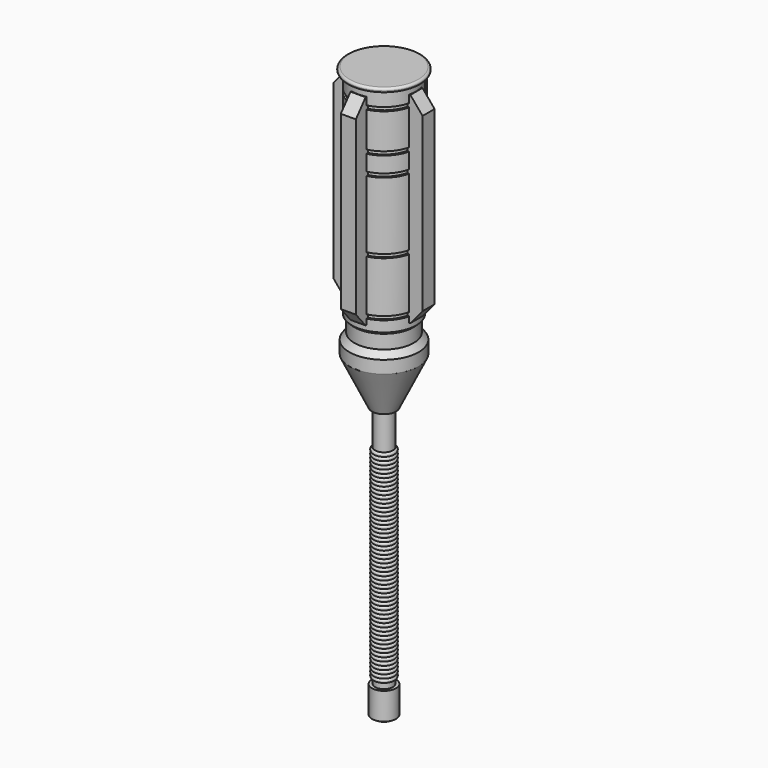
from build123d import *

# Parameters (mm, degrees)
F7_START       = 40
F7_DEPTH       = 31
F10_DEPTH      = 24
F11_COUNT      = 4
F12_R          = 14.2000000015
F13_DEPTH      = 434
F13_DEPTH_BACK = 447.2
F15_START      = -3
F14_R          = 19.2
F14_R_2        = 14.2
F15_DEPTH      = 43
F19_SIZE2      = 4
F19_SIZE       = 4


# Not quite as in the source:
# - ends of sketch curves that miss each other by under 0.0002 mm in the source are joined


with BuildPart() as f2:
    # F0 (on Front) → F2 (revolve)
    with BuildSketch(Plane.XZ):
        Polygon((19.2000000015, -16.7155758262), (55.2000000015, 58.2844241738), (55.2000000015, 78.2844241738), (47.2000000015, 88.5313749398), (47.2000000015, 110.5313749398), (14.2000000015, 110.5313763703), (14.2000000015, -16.7155758262), align=None)
    revolve(axis=Axis((0, 0, 23.2442431152), (0, 0, 1)))


with BuildPart() as f5:
    # F3 (on Front) → F5 (revolve)
    with BuildSketch(Plane.XZ):
        with BuildLine():
            Line((51.2, 112.0996549726), (51.2, 113.5313748121))
            Line((51.2, 113.5313748121), (51.2, 131.5313748121))
            Line((51.2, 131.5313748121), (48.2, 131.5313748121))
            Line((48.2, 131.5313748121), (48.2, 137.5313748121))
            Line((48.2, 137.5313748121), (51.2, 137.5313748121))
            Line((51.2, 137.5313748121), (51.2, 218.5313748121))
            Line((51.2, 218.5313748121), (48.2, 218.5313748121))
            Line((48.2, 218.5313748121), (48.2, 224.5313748121))
            Line((48.2, 224.5313748121), (51.2, 224.5313748121))
            Line((51.2, 224.5313748121), (51.2, 331.5313748121))
            Line((51.2, 331.5313748121), (48.2, 331.5313748121))
            Line((48.2, 331.5313748121), (48.2, 337.5313748121))
            Line((48.2, 337.5313748121), (51.2, 337.5313748121))
            Line((51.2, 337.5313748121), (51.2, 362.5313748121))
            Line((51.2, 362.5313748121), (48.2, 362.5313748121))
            Line((48.2, 362.5313748121), (48.2, 368.5313748121))
            Line((48.2, 368.5313748121), (51.2, 368.5313748121))
            Line((51.2, 368.5313748121), (51.2, 424.5313748121))
            Line((51.2, 424.5313748121), (48.2, 424.5313748121))
            Line((48.2, 424.5313748121), (48.2, 430.5313748121))
            Line((48.2, 430.5313748121), (51.2, 430.5313748121))
            Line((51.2, 430.5313748121), (51.2, 453.5313748121))
            Line((51.2, 453.5313748121), (54.7, 453.5313748121))
            ThreePointArc((54.7, 453.5313748121), (57.1748737342, 454.556501078), (58.2, 457.0313748121))
            ThreePointArc((58.2, 457.0313748121), (57.1748737342, 459.5062485463), (54.7, 460.5313748121))
            Line((54.7, 460.5313748121), (14.2, 460.5313748121))
            Line((14.2, 460.5313748121), (0, 460.5313748121))
            Line((0, 460.5313748121), (0, 430.5313748121))
            Line((0, 430.5313748121), (14.2, 430.5313748121))
            Line((14.2, 430.5313748121), (14.2, 110.5313748121))
            Line((14.2, 110.5313748121), (15.9806390532, 110.5313748121))
            Line((15.9806390532, 110.5313748121), (40.9627765536, 110.5313748121))
            Line((40.9627765536, 110.5313748121), (51.2, 110.5313748121))
            Line((51.2, 110.5313748121), (51.2, 112.0996549726))
        make_face()
    revolve(axis=Axis((0, 0, 255.8234632015), (0, 0, 1)))

    # F19
    f19_edges = [f5.edges().sort_by_distance(p)[0] for p in [
        (-51.2, 0, 110.531375),
    ]]
    chamfer(f19_edges, length=F19_SIZE, length2=F19_SIZE2)


with BuildPart() as f7:
    # F6 (on Front) → F7 (new body)
    with BuildSketch(Plane.XZ.offset(F7_START)):
        Polygon((-12, 122.600607574), (0, 122.600607574), (12, 122.600607574), (12, 442.600607574), (-12, 442.600607574), align=None)
    extrude(amount=F7_DEPTH)

    # F9 (on face) → F10 (cut, through all)
    with BuildSketch(Plane.YZ.offset(12)):
        Polygon((-71, 419.500607574), (-51.6167985198, 442.600607574), (-71, 442.600607574), align=None)
        Polygon((-51.6167985198, 122.600607574), (-71, 145.700607574), (-71, 122.600607574), align=None)
    extrude(amount=-F10_DEPTH, mode=Mode.SUBTRACT)


with BuildPart() as f11_1:
    # F11: instance of F7
    add(f7.part.rotate(Axis((0, 0, 22.6825606078), (0, 0, 1)), 1 * 360 / F11_COUNT))


with BuildPart() as f11_2:
    # F11: instance of F7
    add(f7.part.rotate(Axis((0, 0, 22.6825606078), (0, 0, 1)), 2 * 360 / F11_COUNT))


with BuildPart() as f11_3:
    # F11: instance of F7
    add(f7.part.rotate(Axis((0, 0, 22.6825606078), (0, 0, 1)), 3 * 360 / F11_COUNT))


with BuildPart() as f13:
    # F12 (on face) → F13 (new body, two sides)
    with BuildSketch(Plane(origin=(0, 0, -16.7155758262), x_dir=(1, 0, 0), z_dir=(0, 0, -1))) as f13_sk:
        Circle(F12_R)
    extrude(amount=F13_DEPTH)
    extrude(f13_sk.sketch, amount=-F13_DEPTH_BACK)


with BuildPart() as f15:
    # F14 (on face) → F15 (new body)
    with BuildSketch(Plane(origin=(0, 0, -450.7155758262), x_dir=(1, 0, 0), z_dir=(0, 0, -1)).offset(F15_START)):
        Circle(F14_R)
        Circle(F14_R_2, mode=Mode.SUBTRACT)
    extrude(amount=-F15_DEPTH)


with BuildPart() as f18:
    # F16 (on Right) → F18 (revolve)
    with BuildSketch(Plane.YZ):
        with BuildLine():
            Line((14.2000000924, -78.7955758262), (14.2000000924, -78.8155758262))
            ThreePointArc((14.2000000924, -78.8155758262), (14.3224745795, -78.8130747836), (14.4447448574, -78.8055758262))
            ThreePointArc((14.4447448574, -78.8055758262), (14.3224745795, -78.7980768687), (14.2000000924, -78.7955758262))
        make_face()
        with BuildLine():
            ThreePointArc((14.4447448574, -78.8055758262), (14.3224745795, -78.8130747836), (14.2000000924, -78.8155758262))
            Line((14.2000000924, -78.8155758262), (14.2000000924, -84.7755758262))
            ThreePointArc((14.2000000924, -84.7755758262), (14.3224745795, -84.7780768687), (14.4447448574, -84.7855758262))
            ThreePointArc((14.4447448574, -84.7855758262), (17.2000000924, -81.7955758262), (14.4447448574, -78.8055758262))
        make_face()
        with BuildLine():
            ThreePointArc((14.2000000924, -78.7955758262), (14.3224745795, -78.7980768687), (14.4447448574, -78.8055758262))
            ThreePointArc((14.4447448574, -78.8055758262), (17.1974990499, -75.693101339), (14.2000000924, -72.8155758262))
            Line((14.2000000924, -72.8155758262), (14.2000000924, -78.7955758262))
        make_face()
        with BuildLine():
            ThreePointArc((14.4447448574, -84.7855758262), (14.3224745795, -84.7780768687), (14.2000000924, -84.7755758262))
            Line((14.2000000924, -84.7755758262), (14.2000000924, -84.7955758262))
            ThreePointArc((14.2000000924, -84.7955758262), (14.3224745795, -84.7930747836), (14.4447448574, -84.7855758262))
        make_face()
        with BuildLine():
            ThreePointArc((14.4447448574, -90.7655758262), (17.2000000924, -87.7755758262), (14.4447448574, -84.7855758262))
            ThreePointArc((14.4447448574, -84.7855758262), (14.3224745795, -84.7930747836), (14.2000000924, -84.7955758262))
            Line((14.2000000924, -84.7955758262), (14.2000000924, -90.7555758262))
            ThreePointArc((14.2000000924, -90.7555758262), (14.3224745795, -90.7580768687), (14.4447448574, -90.7655758262))
        make_face()
        with BuildLine():
            ThreePointArc((14.4447448574, -96.7455758262), (17.2000000924, -93.7555758262), (14.4447448574, -90.7655758262))
            ThreePointArc((14.4447448574, -90.7655758262), (14.3224745795, -90.7730747836), (14.2000000924, -90.7755758262))
            Line((14.2000000924, -90.7755758262), (14.2000000924, -96.7355758262))
            ThreePointArc((14.2000000924, -96.7355758262), (14.3224745795, -96.7380768687), (14.4447448574, -96.7455758262))
        make_face()
        with BuildLine():
            ThreePointArc((14.2000000924, -90.7755758262), (14.3224745795, -90.7730747836), (14.4447448574, -90.7655758262))
            ThreePointArc((14.4447448574, -90.7655758262), (14.3224745795, -90.7580768687), (14.2000000924, -90.7555758262))
            Line((14.2000000924, -90.7555758262), (14.2000000924, -90.7755758262))
        make_face()
        with BuildLine():
            ThreePointArc((14.4447448574, -102.7255758262), (17.2000000924, -99.7355758262), (14.4447448574, -96.7455758262))
            ThreePointArc((14.4447448574, -96.7455758262), (14.3224745795, -96.7530747836), (14.2000000924, -96.7555758262))
            Line((14.2000000924, -96.7555758262), (14.2000000924, -102.7155758262))
            ThreePointArc((14.2000000924, -102.7155758262), (14.3224745795, -102.7180768687), (14.4447448574, -102.7255758262))
        make_face()
        with BuildLine():
            ThreePointArc((14.2000000924, -96.7555758262), (14.3224745795, -96.7530747836), (14.4447448574, -96.7455758262))
            ThreePointArc((14.4447448574, -96.7455758262), (14.3224745795, -96.7380768687), (14.2000000924, -96.7355758262))
            Line((14.2000000924, -96.7355758262), (14.2000000924, -96.7555758262))
        make_face()
        with BuildLine():
            ThreePointArc((14.4447448574, -108.7055758262), (17.2000000924, -105.7155758262), (14.4447448574, -102.7255758262))
            ThreePointArc((14.4447448574, -102.7255758262), (14.3224745795, -102.7330747836), (14.2000000924, -102.7355758262))
            Line((14.2000000924, -102.7355758262), (14.2000000924, -108.6955758262))
            ThreePointArc((14.2000000924, -108.6955758262), (14.3224745795, -108.6980768687), (14.4447448574, -108.7055758262))
        make_face()
        with BuildLine():
            ThreePointArc((14.2000000924, -102.7355758262), (14.3224745795, -102.7330747836), (14.4447448574, -102.7255758262))
            ThreePointArc((14.4447448574, -102.7255758262), (14.3224745795, -102.7180768687), (14.2000000924, -102.7155758262))
            Line((14.2000000924, -102.7155758262), (14.2000000924, -102.7355758262))
        make_face()
        with BuildLine():
            ThreePointArc((14.4447448574, -114.6855758262), (17.2000000924, -111.6955758262), (14.4447448574, -108.7055758262))
            ThreePointArc((14.4447448574, -108.7055758262), (14.3224745795, -108.7130747836), (14.2000000924, -108.7155758262))
            Line((14.2000000924, -108.7155758262), (14.2000000924, -114.6755758262))
            ThreePointArc((14.2000000924, -114.6755758262), (14.3224745795, -114.6780768687), (14.4447448574, -114.6855758262))
        make_face()
        with BuildLine():
            ThreePointArc((14.2000000924, -108.7155758262), (14.3224745795, -108.7130747836), (14.4447448574, -108.7055758262))
            ThreePointArc((14.4447448574, -108.7055758262), (14.3224745795, -108.6980768687), (14.2000000924, -108.6955758262))
            Line((14.2000000924, -108.6955758262), (14.2000000924, -108.7155758262))
        make_face()
        with BuildLine():
            ThreePointArc((14.4447448574, -120.6655758262), (17.2000000924, -117.6755758262), (14.4447448574, -114.6855758262))
            ThreePointArc((14.4447448574, -114.6855758262), (14.3224745795, -114.6930747836), (14.2000000924, -114.6955758262))
            Line((14.2000000924, -114.6955758262), (14.2000000924, -120.6555758262))
            ThreePointArc((14.2000000924, -120.6555758262), (14.3224745795, -120.6580768687), (14.4447448574, -120.6655758262))
        make_face()
        with BuildLine():
            ThreePointArc((14.2000000924, -114.6955758262), (14.3224745795, -114.6930747836), (14.4447448574, -114.6855758262))
            ThreePointArc((14.4447448574, -114.6855758262), (14.3224745795, -114.6780768687), (14.2000000924, -114.6755758262))
            Line((14.2000000924, -114.6755758262), (14.2000000924, -114.6955758262))
        make_face()
        with BuildLine():
            ThreePointArc((14.4447448574, -126.6455758262), (17.2000000924, -123.6555758262), (14.4447448574, -120.6655758262))
            ThreePointArc((14.4447448574, -120.6655758262), (14.3224745795, -120.6730747836), (14.2000000924, -120.6755758262))
            Line((14.2000000924, -120.6755758262), (14.2000000924, -126.6355758262))
            ThreePointArc((14.2000000924, -126.6355758262), (14.3224745795, -126.6380768687), (14.4447448574, -126.6455758262))
        make_face()
        with BuildLine():
            ThreePointArc((14.2000000924, -120.6755758262), (14.3224745795, -120.6730747836), (14.4447448574, -120.6655758262))
            ThreePointArc((14.4447448574, -120.6655758262), (14.3224745795, -120.6580768687), (14.2000000924, -120.6555758262))
            Line((14.2000000924, -120.6555758262), (14.2000000924, -120.6755758262))
        make_face()
        with BuildLine():
            ThreePointArc((14.4447448574, -132.6255758262), (17.2000000924, -129.6355758262), (14.4447448574, -126.6455758262))
            ThreePointArc((14.4447448574, -126.6455758262), (14.3224745795, -126.6530747836), (14.2000000924, -126.6555758262))
            Line((14.2000000924, -126.6555758262), (14.2000000924, -132.6155758262))
            ThreePointArc((14.2000000924, -132.6155758262), (14.3224745795, -132.6180768687), (14.4447448574, -132.6255758262))
        make_face()
        with BuildLine():
            ThreePointArc((14.2000000924, -126.6555758262), (14.3224745795, -126.6530747836), (14.4447448574, -126.6455758262))
            ThreePointArc((14.4447448574, -126.6455758262), (14.3224745795, -126.6380768687), (14.2000000924, -126.6355758262))
            Line((14.2000000924, -126.6355758262), (14.2000000924, -126.6555758262))
        make_face()
        with BuildLine():
            ThreePointArc((14.4447448574, -138.6055758262), (17.2000000924, -135.6155758262), (14.4447448574, -132.6255758262))
            ThreePointArc((14.4447448574, -132.6255758262), (14.3224745795, -132.6330747836), (14.2000000924, -132.6355758262))
            Line((14.2000000924, -132.6355758262), (14.2000000924, -138.5955758262))
            ThreePointArc((14.2000000924, -138.5955758262), (14.3224745795, -138.5980768687), (14.4447448574, -138.6055758262))
        make_face()
        with BuildLine():
            ThreePointArc((14.2000000924, -132.6355758262), (14.3224745795, -132.6330747836), (14.4447448574, -132.6255758262))
            ThreePointArc((14.4447448574, -132.6255758262), (14.3224745795, -132.6180768687), (14.2000000924, -132.6155758262))
            Line((14.2000000924, -132.6155758262), (14.2000000924, -132.6355758262))
        make_face()
        with BuildLine():
            ThreePointArc((14.4447448574, -144.5855758262), (17.2000000924, -141.5955758262), (14.4447448574, -138.6055758262))
            ThreePointArc((14.4447448574, -138.6055758262), (14.3224745795, -138.6130747836), (14.2000000924, -138.6155758262))
            Line((14.2000000924, -138.6155758262), (14.2000000924, -144.5755758262))
            ThreePointArc((14.2000000924, -144.5755758262), (14.3224745795, -144.5780768687), (14.4447448574, -144.5855758262))
        make_face()
        with BuildLine():
            ThreePointArc((14.2000000924, -138.6155758262), (14.3224745795, -138.6130747836), (14.4447448574, -138.6055758262))
            ThreePointArc((14.4447448574, -138.6055758262), (14.3224745795, -138.5980768687), (14.2000000924, -138.5955758262))
            Line((14.2000000924, -138.5955758262), (14.2000000924, -138.6155758262))
        make_face()
        with BuildLine():
            ThreePointArc((14.4447448574, -150.5655758262), (17.2000000924, -147.5755758262), (14.4447448574, -144.5855758262))
            ThreePointArc((14.4447448574, -144.5855758262), (14.3224745795, -144.5930747836), (14.2000000924, -144.5955758262))
            Line((14.2000000924, -144.5955758262), (14.2000000924, -150.5555758262))
            ThreePointArc((14.2000000924, -150.5555758262), (14.3224745795, -150.5580768687), (14.4447448574, -150.5655758262))
        make_face()
        with BuildLine():
            ThreePointArc((14.2000000924, -144.5955758262), (14.3224745795, -144.5930747836), (14.4447448574, -144.5855758262))
            ThreePointArc((14.4447448574, -144.5855758262), (14.3224745795, -144.5780768687), (14.2000000924, -144.5755758262))
            Line((14.2000000924, -144.5755758262), (14.2000000924, -144.5955758262))
        make_face()
        with BuildLine():
            ThreePointArc((14.4447448574, -156.5455758262), (17.2000000924, -153.5555758262), (14.4447448574, -150.5655758262))
            ThreePointArc((14.4447448574, -150.5655758262), (14.3224745795, -150.5730747836), (14.2000000924, -150.5755758262))
            Line((14.2000000924, -150.5755758262), (14.2000000924, -156.5355758262))
            ThreePointArc((14.2000000924, -156.5355758262), (14.3224745795, -156.5380768687), (14.4447448574, -156.5455758262))
        make_face()
        with BuildLine():
            ThreePointArc((14.2000000924, -150.5755758262), (14.3224745795, -150.5730747836), (14.4447448574, -150.5655758262))
            ThreePointArc((14.4447448574, -150.5655758262), (14.3224745795, -150.5580768687), (14.2000000924, -150.5555758262))
            Line((14.2000000924, -150.5555758262), (14.2000000924, -150.5755758262))
        make_face()
        with BuildLine():
            ThreePointArc((14.4447448574, -162.5255758262), (17.2000000924, -159.5355758262), (14.4447448574, -156.5455758262))
            ThreePointArc((14.4447448574, -156.5455758262), (14.3224745795, -156.5530747836), (14.2000000924, -156.5555758262))
            Line((14.2000000924, -156.5555758262), (14.2000000924, -162.5155758262))
            ThreePointArc((14.2000000924, -162.5155758262), (14.3224745795, -162.5180768687), (14.4447448574, -162.5255758262))
        make_face()
        with BuildLine():
            ThreePointArc((14.2000000924, -156.5555758262), (14.3224745795, -156.5530747836), (14.4447448574, -156.5455758262))
            ThreePointArc((14.4447448574, -156.5455758262), (14.3224745795, -156.5380768687), (14.2000000924, -156.5355758262))
            Line((14.2000000924, -156.5355758262), (14.2000000924, -156.5555758262))
        make_face()
        with BuildLine():
            ThreePointArc((14.4447448574, -168.5055758262), (17.2000000924, -165.5155758262), (14.4447448574, -162.5255758262))
            ThreePointArc((14.4447448574, -162.5255758262), (14.3224745795, -162.5330747836), (14.2000000924, -162.5355758262))
            Line((14.2000000924, -162.5355758262), (14.2000000924, -168.4955758262))
            ThreePointArc((14.2000000924, -168.4955758262), (14.3224745795, -168.4980768687), (14.4447448574, -168.5055758262))
        make_face()
        with BuildLine():
            ThreePointArc((14.2000000924, -162.5355758262), (14.3224745795, -162.5330747836), (14.4447448574, -162.5255758262))
            ThreePointArc((14.4447448574, -162.5255758262), (14.3224745795, -162.5180768687), (14.2000000924, -162.5155758262))
            Line((14.2000000924, -162.5155758262), (14.2000000924, -162.5355758262))
        make_face()
        with BuildLine():
            ThreePointArc((14.4447448574, -174.4855758262), (17.2000000924, -171.4955758262), (14.4447448574, -168.5055758262))
            ThreePointArc((14.4447448574, -168.5055758262), (14.3224745795, -168.5130747836), (14.2000000924, -168.5155758262))
            Line((14.2000000924, -168.5155758262), (14.2000000924, -174.4755758262))
            ThreePointArc((14.2000000924, -174.4755758262), (14.3224745795, -174.4780768687), (14.4447448574, -174.4855758262))
        make_face()
        with BuildLine():
            ThreePointArc((14.2000000924, -168.5155758262), (14.3224745795, -168.5130747836), (14.4447448574, -168.5055758262))
            ThreePointArc((14.4447448574, -168.5055758262), (14.3224745795, -168.4980768687), (14.2000000924, -168.4955758262))
            Line((14.2000000924, -168.4955758262), (14.2000000924, -168.5155758262))
        make_face()
        with BuildLine():
            ThreePointArc((14.4447448574, -180.4655758262), (17.2000000924, -177.4755758262), (14.4447448574, -174.4855758262))
            ThreePointArc((14.4447448574, -174.4855758262), (14.3224745795, -174.4930747836), (14.2000000924, -174.4955758262))
            Line((14.2000000924, -174.4955758262), (14.2000000924, -180.4555758262))
            ThreePointArc((14.2000000924, -180.4555758262), (14.3224745795, -180.4580768687), (14.4447448574, -180.4655758262))
        make_face()
        with BuildLine():
            ThreePointArc((14.2000000924, -174.4955758262), (14.3224745795, -174.4930747836), (14.4447448574, -174.4855758262))
            ThreePointArc((14.4447448574, -174.4855758262), (14.3224745795, -174.4780768687), (14.2000000924, -174.4755758262))
            Line((14.2000000924, -174.4755758262), (14.2000000924, -174.4955758262))
        make_face()
        with BuildLine():
            ThreePointArc((14.4447448574, -186.4455758262), (17.2000000924, -183.4555758262), (14.4447448574, -180.4655758262))
            ThreePointArc((14.4447448574, -180.4655758262), (14.3224745795, -180.4730747836), (14.2000000924, -180.4755758262))
            Line((14.2000000924, -180.4755758262), (14.2000000924, -186.4355758262))
            ThreePointArc((14.2000000924, -186.4355758262), (14.3224745795, -186.4380768687), (14.4447448574, -186.4455758262))
        make_face()
        with BuildLine():
            ThreePointArc((14.2000000924, -180.4755758262), (14.3224745795, -180.4730747836), (14.4447448574, -180.4655758262))
            ThreePointArc((14.4447448574, -180.4655758262), (14.3224745795, -180.4580768687), (14.2000000924, -180.4555758262))
            Line((14.2000000924, -180.4555758262), (14.2000000924, -180.4755758262))
        make_face()
        with BuildLine():
            ThreePointArc((14.4447448574, -192.4255758262), (17.2000000924, -189.4355758262), (14.4447448574, -186.4455758262))
            ThreePointArc((14.4447448574, -186.4455758262), (14.3224745795, -186.4530747836), (14.2000000924, -186.4555758262))
            Line((14.2000000924, -186.4555758262), (14.2000000924, -192.4155758262))
            ThreePointArc((14.2000000924, -192.4155758262), (14.3224745795, -192.4180768687), (14.4447448574, -192.4255758262))
        make_face()
        with BuildLine():
            ThreePointArc((14.2000000924, -186.4555758262), (14.3224745795, -186.4530747836), (14.4447448574, -186.4455758262))
            ThreePointArc((14.4447448574, -186.4455758262), (14.3224745795, -186.4380768687), (14.2000000924, -186.4355758262))
            Line((14.2000000924, -186.4355758262), (14.2000000924, -186.4555758262))
        make_face()
        with BuildLine():
            ThreePointArc((14.4447448574, -198.4055758262), (17.2000000924, -195.4155758262), (14.4447448574, -192.4255758262))
            ThreePointArc((14.4447448574, -192.4255758262), (14.3224745795, -192.4330747836), (14.2000000924, -192.4355758262))
            Line((14.2000000924, -192.4355758262), (14.2000000924, -198.3955758262))
            ThreePointArc((14.2000000924, -198.3955758262), (14.3224745795, -198.3980768687), (14.4447448574, -198.4055758262))
        make_face()
        with BuildLine():
            ThreePointArc((14.2000000924, -192.4355758262), (14.3224745795, -192.4330747836), (14.4447448574, -192.4255758262))
            ThreePointArc((14.4447448574, -192.4255758262), (14.3224745795, -192.4180768687), (14.2000000924, -192.4155758262))
            Line((14.2000000924, -192.4155758262), (14.2000000924, -192.4355758262))
        make_face()
        with BuildLine():
            ThreePointArc((14.4447448574, -204.3855758262), (17.2000000924, -201.3955758262), (14.4447448574, -198.4055758262))
            ThreePointArc((14.4447448574, -198.4055758262), (14.3224745795, -198.4130747836), (14.2000000924, -198.4155758262))
            Line((14.2000000924, -198.4155758262), (14.2000000924, -204.3755758262))
            ThreePointArc((14.2000000924, -204.3755758262), (14.3224745795, -204.3780768687), (14.4447448574, -204.3855758262))
        make_face()
        with BuildLine():
            ThreePointArc((14.2000000924, -198.4155758262), (14.3224745795, -198.4130747836), (14.4447448574, -198.4055758262))
            ThreePointArc((14.4447448574, -198.4055758262), (14.3224745795, -198.3980768687), (14.2000000924, -198.3955758262))
            Line((14.2000000924, -198.3955758262), (14.2000000924, -198.4155758262))
        make_face()
        with BuildLine():
            ThreePointArc((14.4447448574, -210.3655758262), (17.2000000924, -207.3755758262), (14.4447448574, -204.3855758262))
            ThreePointArc((14.4447448574, -204.3855758262), (14.3224745795, -204.3930747836), (14.2000000924, -204.3955758262))
            Line((14.2000000924, -204.3955758262), (14.2000000924, -210.3555758262))
            ThreePointArc((14.2000000924, -210.3555758262), (14.3224745795, -210.3580768687), (14.4447448574, -210.3655758262))
        make_face()
        with BuildLine():
            ThreePointArc((14.2000000924, -204.3955758262), (14.3224745795, -204.3930747836), (14.4447448574, -204.3855758262))
            ThreePointArc((14.4447448574, -204.3855758262), (14.3224745795, -204.3780768687), (14.2000000924, -204.3755758262))
            Line((14.2000000924, -204.3755758262), (14.2000000924, -204.3955758262))
        make_face()
        with BuildLine():
            ThreePointArc((14.4447448574, -216.3455758262), (17.2000000924, -213.3555758262), (14.4447448574, -210.3655758262))
            ThreePointArc((14.4447448574, -210.3655758262), (14.3224745795, -210.3730747836), (14.2000000924, -210.3755758262))
            Line((14.2000000924, -210.3755758262), (14.2000000924, -216.3355758262))
            ThreePointArc((14.2000000924, -216.3355758262), (14.3224745795, -216.3380768687), (14.4447448574, -216.3455758262))
        make_face()
        with BuildLine():
            ThreePointArc((14.2000000924, -210.3755758262), (14.3224745795, -210.3730747836), (14.4447448574, -210.3655758262))
            ThreePointArc((14.4447448574, -210.3655758262), (14.3224745795, -210.3580768687), (14.2000000924, -210.3555758262))
            Line((14.2000000924, -210.3555758262), (14.2000000924, -210.3755758262))
        make_face()
        with BuildLine():
            ThreePointArc((14.4447448574, -222.3255758262), (17.2000000924, -219.3355758262), (14.4447448574, -216.3455758262))
            ThreePointArc((14.4447448574, -216.3455758262), (14.3224745795, -216.3530747836), (14.2000000924, -216.3555758262))
            Line((14.2000000924, -216.3555758262), (14.2000000924, -222.3155758262))
            ThreePointArc((14.2000000924, -222.3155758262), (14.3224745795, -222.3180768687), (14.4447448574, -222.3255758262))
        make_face()
        with BuildLine():
            ThreePointArc((14.2000000924, -216.3555758262), (14.3224745795, -216.3530747836), (14.4447448574, -216.3455758262))
            ThreePointArc((14.4447448574, -216.3455758262), (14.3224745795, -216.3380768687), (14.2000000924, -216.3355758262))
            Line((14.2000000924, -216.3355758262), (14.2000000924, -216.3555758262))
        make_face()
        with BuildLine():
            ThreePointArc((14.4447448574, -228.3055758262), (17.2000000924, -225.3155758262), (14.4447448574, -222.3255758262))
            ThreePointArc((14.4447448574, -222.3255758262), (14.3224745795, -222.3330747836), (14.2000000924, -222.3355758262))
            Line((14.2000000924, -222.3355758262), (14.2000000924, -228.2955758262))
            ThreePointArc((14.2000000924, -228.2955758262), (14.3224745795, -228.2980768687), (14.4447448574, -228.3055758262))
        make_face()
        with BuildLine():
            ThreePointArc((14.2000000924, -222.3355758262), (14.3224745795, -222.3330747836), (14.4447448574, -222.3255758262))
            ThreePointArc((14.4447448574, -222.3255758262), (14.3224745795, -222.3180768687), (14.2000000924, -222.3155758262))
            Line((14.2000000924, -222.3155758262), (14.2000000924, -222.3355758262))
        make_face()
        with BuildLine():
            ThreePointArc((14.2000000924, -234.2955758262), (17.1974990499, -231.4180503133), (14.4447448574, -228.3055758262))
            ThreePointArc((14.4447448574, -228.3055758262), (14.3224745795, -228.3130747836), (14.2000000924, -228.3155758262))
            Line((14.2000000924, -228.3155758262), (14.2000000924, -234.2955758262))
        make_face()
        with BuildLine():
            ThreePointArc((14.2000000924, -228.3155758262), (14.3224745795, -228.3130747836), (14.4447448574, -228.3055758262))
            ThreePointArc((14.4447448574, -228.3055758262), (14.3224745795, -228.2980768687), (14.2000000924, -228.2955758262))
            Line((14.2000000924, -228.2955758262), (14.2000000924, -228.3155758262))
        make_face()
    revolve(axis=Axis((0, 0, -20.6363089383), (0, 0, -1)))


with BuildPart() as f21_1:
    # F21: instance of F18
    add(f18.part.mirror(Plane(origin=(0, 0, -234.2955758262), x_dir=(1, 0, 0), z_dir=(0, 0, -1))))


solid = Compound([f2.part, f5.part, f7.part, f11_1.part, f11_2.part, f11_3.part, f13.part, f15.part, f18.part, f21_1.part])
